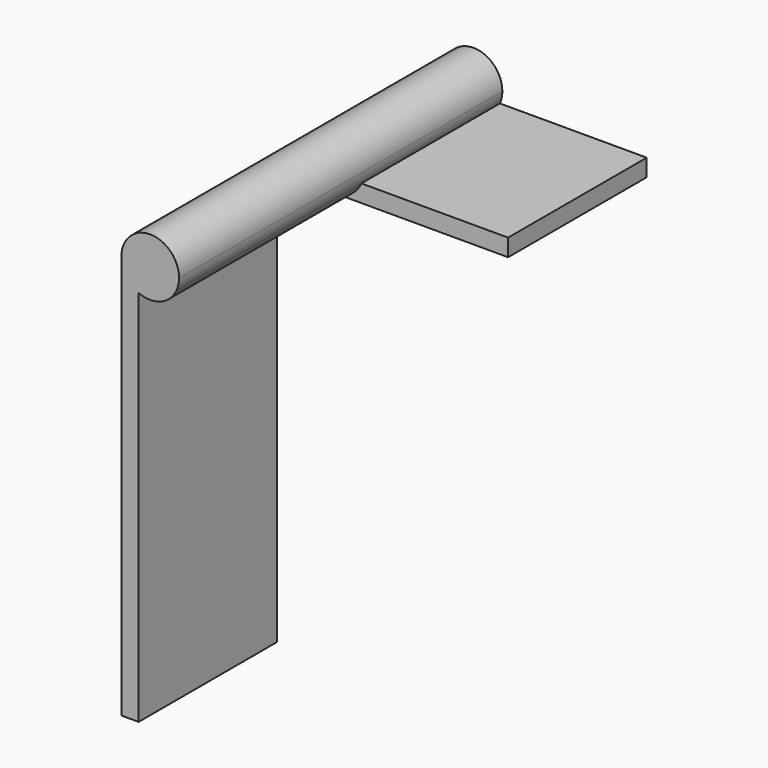
from build123d import *

# Parameters (mm, degrees)
F1_DEPTH = 70
F2_DEPTH = 30
F4_DEPTH = 30


# Not quite as in the source:
# - a feature names something its author has since deleted; it is built from what else it names


with BuildPart() as f1:
    # F0 (on Front) → F1 (new body)
    with BuildSketch(Plane.XZ):
        with BuildLine():
            ThreePointArc((4.582575695, -2), (4.8945315647, -1.0215482184), (5, 0))
            ThreePointArc((5, 0), (-3.5355339059, 3.5355339059), (0, -5))
            Line((0, -5), (0, -2))
            Line((0, -2), (4.582575695, -2))
        make_face()
        with BuildLine():
            Line((0, -2), (0, -5))
            ThreePointArc((0, -5), (2.7386127875, -4.1833001327), (4.582575695, -2))
            Line((4.582575695, -2), (0, -2))
        make_face()
    extrude(amount=F1_DEPTH)

    # F0 (on Front) → F2 (join)
    with BuildSketch(Plane.XZ):
        with BuildLine():
            ThreePointArc((4.582575695, -2), (2.7386127875, -4.1833001327), (0, -5))
            Line((0, -5), (30, -5))
            Line((30, -5), (30, -2))
            Line((30, -2), (4.582575695, -2))
        make_face()
    extrude(amount=F2_DEPTH)

    # F3 (on face) → F4 (join)
    with BuildSketch(Plane.XZ.offset(70)):
        with BuildLine():
            Line((-2, -70), (-2, -4.582575695))
            ThreePointArc((-2, -4.582575695), (-4.1833001327, -2.7386127875), (-5, 0))
            Line((-5, 0), (-5, -70))
            Line((-5, -70), (-2, -70))
        make_face()
    extrude(amount=-F4_DEPTH)


solid = f1.part
